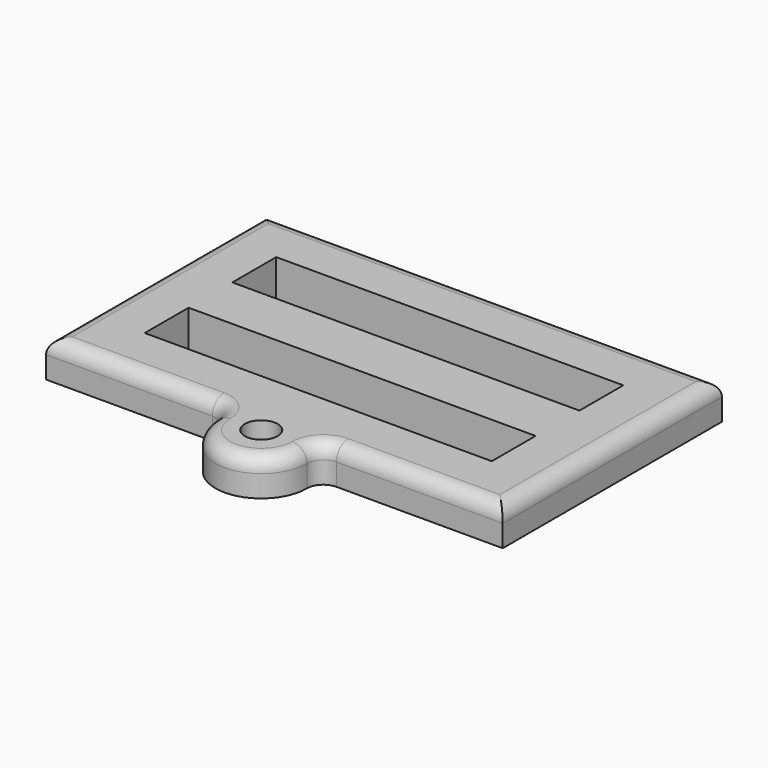
from build123d import *

# Parameters (mm, degrees)
F0_R     = 0.9
F0_W     = 19
F0_H     = 3
F1_DEPTH = 2
F2_R     = 0.89999
F3_R     = 0.8


# Not quite as in the source:
# - a fillet or chamfer is up to 0.001 mm smaller than in the source, because OpenCascade refuses the exact size


with BuildPart() as f1:
    # F0 (on Top) → F1 (new body)
    with BuildSketch(Plane.XY):
        with BuildLine():
            Line((12.5, 7.5), (-12.5, 7.5))
            Line((-12.5, 7.5), (-12.5, -7.5))
            Line((-12.5, -7.5), (-2.5, -7.5))
            Line((-2.5, -7.5), (-2.5, -8.4))
            ThreePointArc((-2.5, -8.4), (0, -10.9), (2.5, -8.4))
            Line((2.5, -8.4), (2.5, -7.5))
            Line((2.5, -7.5), (12.5, -7.5))
            Line((12.5, -7.5), (12.5, 7.5))
        make_face()
        with Locations((0, -8.4)):
            Circle(F0_R, mode=Mode.SUBTRACT)
        with Locations((0, -3)):
            Rectangle(F0_W, F0_H, mode=Mode.SUBTRACT)
        with Locations((0, 3)):
            Rectangle(F0_W, F0_H, mode=Mode.SUBTRACT)
    extrude(amount=F1_DEPTH)

    # F2 (radius 0.9 in the source; OpenCascade refuses exactly that, so slightly less here)
    f2_edges = [f1.edges().sort_by_distance(p)[0] for p in [
        (2.5, -7.5, 1),
        (-2.5, -7.5, 1),
    ]]
    fillet(f2_edges, radius=F2_R)

    # F3
    f3_edges = [f1.edges().sort_by_distance(p)[0] for p in [
        (12.5, 0, 2),
        (7.949995, -7.5, 2),
        (-12.5, 0, 2),
        (0, 7.5, 2),
    ]]
    fillet(f3_edges, radius=F3_R)


solid = f1.part
